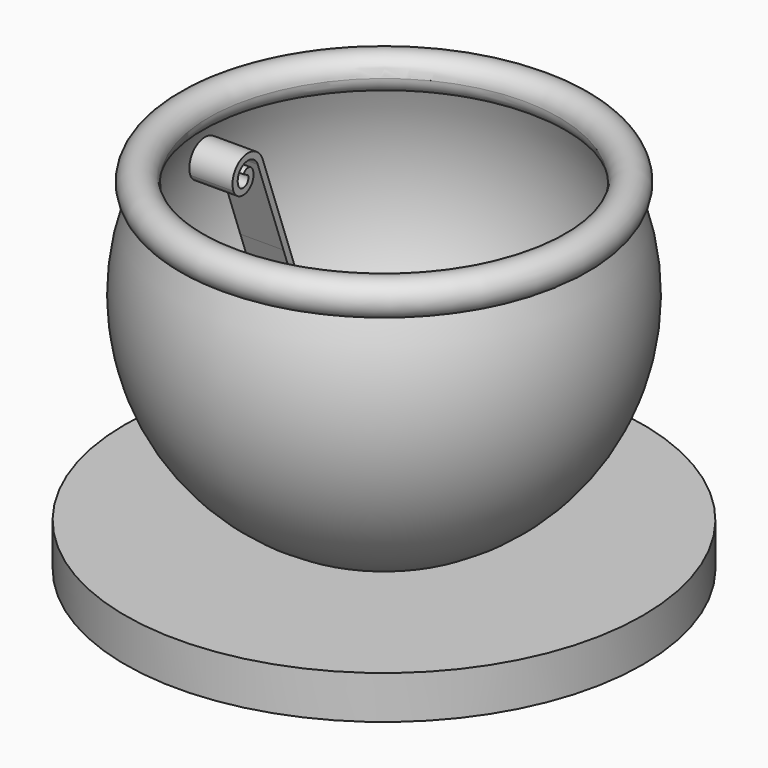
from build123d import *

# Parameters (mm, degrees)
F0_R     = 38.1
F1_DEPTH = 6.35
F6_R     = 2.54
F9_DEPTH = 3.175


# Not quite as in the source:
# - a feature of the source that left no trace in its solid (it failed there, or was rolled back) is left out


with BuildPart() as f1:
    # F0 (on Top) → F1 (new body)
    with BuildSketch(Plane.XY):
        Circle(F0_R)
    extrude(amount=F1_DEPTH)

    # F2 (on Right) → F3 (revolve)
    with BuildSketch(Plane.YZ):
        with BuildLine():
            Line((-12.7, 6.35), (0, 6.35))
            Line((0, 6.35), (0, 35.56))
            Line((0, 35.56), (0, 50.165))
            Line((0, 50.165), (-28.3056191418, 50.165))
            ThreePointArc((-28.3056191418, 50.165), (-30.0050621821, 24.873076053), (-12.7, 6.35))
        make_face()
    revolve(axis=Axis((0, 0, 20.955), (0, 0, 1)))

    # F4 (on Right) → F5 (revolve, cut)
    with BuildSketch(Plane.YZ):
        with BuildLine():
            Line((0, 50.8879350554), (-26.3454893091, 50.8879350554))
            ThreePointArc((-26.3454893091, 50.8879350554), (-26.4218267772, 20.3640311347), (0, 5.08))
            Line((0, 5.08), (0, 50.8879350554))
        make_face()
    revolve(axis=Axis((0, 0, 27.9839675277), (0, 0, 1)), mode=Mode.SUBTRACT)

    # F6 (on Right) → F7 (revolve)
    with BuildSketch(Plane.YZ):
        with Locations((-28.3113475889, 50.1700490713)):
            Circle(F6_R)
    revolve(axis=Axis((0, 0, 42.8625), (0, 0, 1)))


with BuildPart() as f9:
    # F8 (on Right) → F9 (new body, symmetric)
    with BuildSketch(Plane.YZ):
        Polygon((-22.4736384776, 51.5050616825), (-7.2512423155, 9.5923191554), (-6.3559615385, 9.9174784707), (-26.2990662121, 64.828032793), (-27.1943469891, 64.5028734777), align=None)
        with BuildLine():
            ThreePointArc((-30.7754700971, 63.2022362163), (-29.6352271737, 65.643116401), (-27.1943469891, 64.5028734777))
            Line((-27.1943469891, 64.5028734777), (-26.2990662121, 64.828032793))
            ThreePointArc((-26.2990662121, 64.828032793), (-29.9687584763, 66.561448276), (-31.6707508741, 62.877076901))
            ThreePointArc((-31.6707508741, 62.877076901), (-29.2298706894, 61.7368339777), (-28.0896277661, 64.1777141623))
            ThreePointArc((-28.0896277661, 64.1777141623), (-28.9126015709, 64.8245765344), (-29.8222257495, 64.3065990584))
            Line((-29.8222257495, 64.3065990584), (-28.9849085431, 63.852554847))
            ThreePointArc((-28.9849085431, 63.852554847), (-29.5491543746, 62.6159370274), (-30.7754700971, 63.2022362163))
        make_face()
    extrude(amount=F9_DEPTH, both=True)

    # F10 (on Right) → F11 (revolve)
    with BuildSketch(Plane.YZ):
        with BuildLine():
            Line((-6.3914712344, 9.9045816134), (-7.2867520114, 9.5794222981))
            ThreePointArc((-7.2867520114, 9.5794222981), (-4.0057918424, 5.9939412982), (0.8495152707, 5.7786125537))
            Line((0.8495152707, 5.7786125537), (0.5243559554, 6.6738933307))
            ThreePointArc((0.5243559554, 6.6738933307), (-3.6026550908, 6.8569227635), (-6.3914712344, 9.9045816134))
        make_face()
    revolve(axis=Axis((0, -0.3969287714, 9.2105221988), (0, 0.3413746093, -0.9399273249)))


solid = Compound([f1.part, f9.part])
